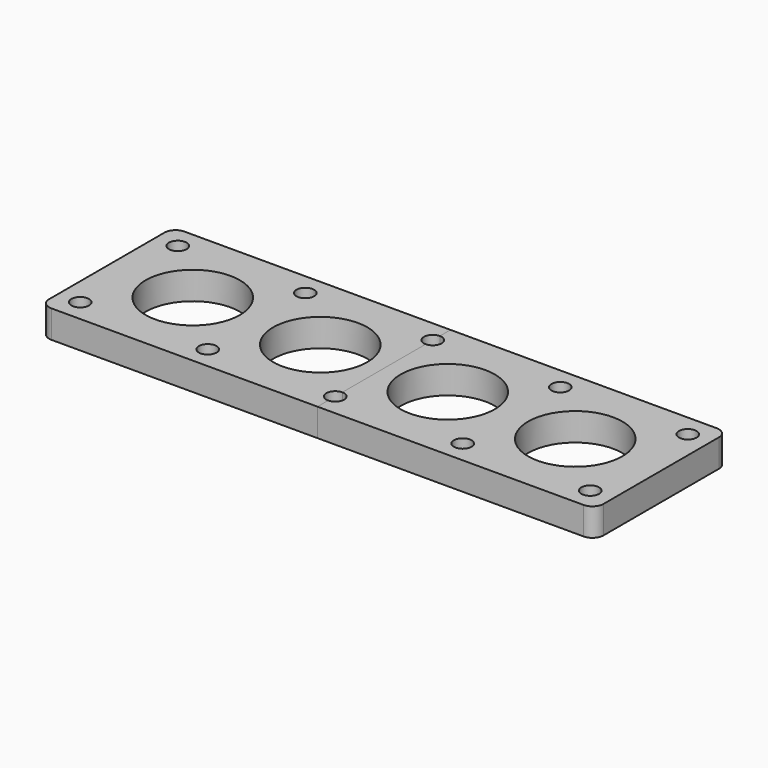
from build123d import *
from build123d import SkipClean  # not in build123d's __all__

# Parameters (mm, degrees)
F2_R     = 8
F2_R_2   = 42.5
F0_DEPTH = 25


with BuildPart() as f0:
    # F2 (on Top) → F0 (new body)
    with BuildSketch(Plane.XY):
        with BuildLine():
            Line((0, -12), (0, 0))
            Line((0, 0), (-240, 0))
            ThreePointArc((-240, 0), (-247.0710678119, -2.9289321881), (-250, -10))
            Line((-250, -10), (-250, -140))
            ThreePointArc((-250, -140), (-247.0710678119, -147.0710678119), (-240, -150))
            Line((-240, -150), (0, -150))
            Line((0, -150), (0, -138))
            ThreePointArc((0, -138), (-8, -130), (0, -122))
            Line((0, -122), (0, -28))
            ThreePointArc((0, -28), (-8, -20), (0, -12))
        make_face()
        with Locations((-230, -130)):
            Circle(F2_R, mode=Mode.SUBTRACT)
        with Locations((-115, -130)):
            Circle(F2_R, mode=Mode.SUBTRACT)
        with Locations((-172.5, -75)):
            Circle(F2_R_2, mode=Mode.SUBTRACT)
        with Locations((-230, -20)):
            Circle(F2_R, mode=Mode.SUBTRACT)
        with Locations((-57.5, -75)):
            Circle(F2_R_2, mode=Mode.SUBTRACT)
        with Locations((-115, -20)):
            Circle(F2_R, mode=Mode.SUBTRACT)
    extrude(amount=F0_DEPTH)

    # F1: F0 across face


with BuildPart() as f0_1:
    add(f0.part, clean=False)
    with SkipClean():  # cleaning this boolean's faces spoils the solid; the shape is the same uncleaned
        add(f0.part.mirror(Plane(origin=(0, -75, 12.5), x_dir=(0, 1, 0), z_dir=(1, 0, 0))), clean=False)


solid = f0_1.part
